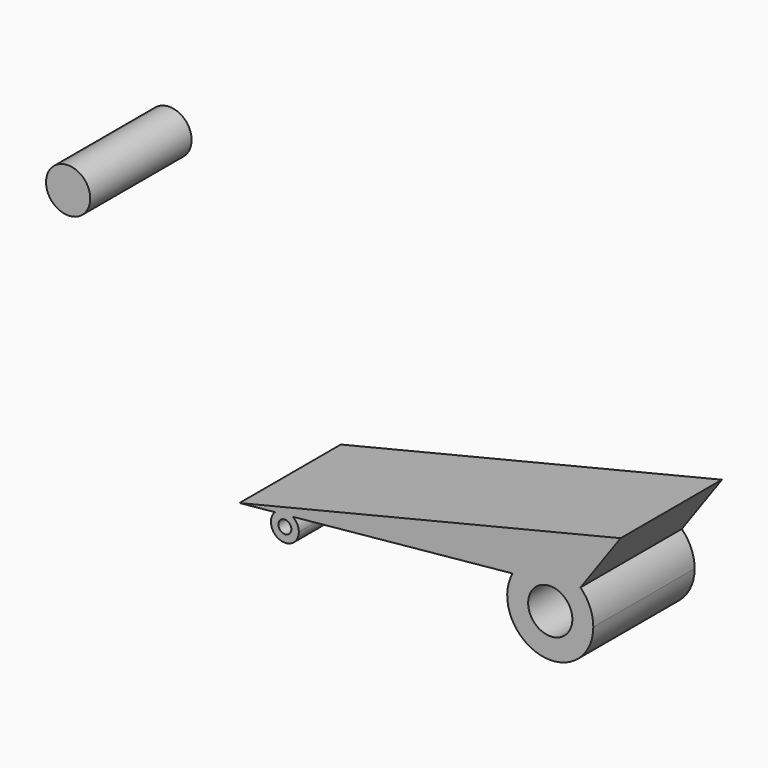
from build123d import *

# Parameters (mm, degrees)
F0_R     = 1.2955888687
F0_R_2   = 4.4335115967
F1_DEPTH = 25.4


with BuildPart() as f1:
    # F0 (on Front) → F1 (new body)
    with BuildSketch(Plane.XZ):
        with BuildLine():
            Line((89.1572237015, 31.5077528358), (12.7428583801, 12.8701059148))
            Line((12.7428583801, 12.8701059148), (19.8439891704, 13.5662951334))
            ThreePointArc((19.8439891704, 13.5662951334), (21.5718320787, 14.3954167349), (23.4278013561, 13.9176492317))
            Line((23.4278013561, 13.9176492317), (67.5118393184, 18.2396132754))
            ThreePointArc((67.5118393184, 18.2396132754), (73.8275336357, 22.5889714613), (81.112807161, 20.1952920757))
            Line((81.112807161, 20.1952920757), (89.1572237015, 31.5077528358))
        make_face()
        with BuildLine():
            ThreePointArc((23.4278013561, 13.9176492317), (21.5718320787, 14.3954167349), (19.8439891704, 13.5662951334))
            Line((19.8439891704, 13.5662951334), (23.4278013561, 13.9176492317))
        make_face()
        with BuildLine():
            Line((23.4278013561, 13.9176492317), (19.8439891704, 13.5662951334))
            ThreePointArc((19.8439891704, 13.5662951334), (20.7894933235, 9.0214762693), (24.6417307995, 11.6117702758))
            ThreePointArc((24.6417307995, 11.6117702758), (24.3197112814, 12.9147190903), (23.4278013561, 13.9176492317))
        make_face()
        with Locations((21.8447385651, 11.6117702758)):
            Circle(F0_R, mode=Mode.SUBTRACT)
        with BuildLine():
            ThreePointArc((83.6881530447, 14.0447923914), (83.0183282504, 17.3787484794), (81.112807161, 20.1952920757))
            Line((81.112807161, 20.1952920757), (80.6371569633, 19.5264089853))
            Line((80.6371569633, 19.5264089853), (67.5118393184, 18.2396132754))
            ThreePointArc((67.5118393184, 18.2396132754), (72.8893138351, 5.6891109706), (83.6881530447, 14.0447923914))
        make_face()
        with Locations((75.0560984015, 14.0447923914)):
            Circle(F0_R_2, mode=Mode.SUBTRACT)
        with BuildLine():
            Line((80.6371569633, 19.5264089853), (81.112807161, 20.1952920757))
            ThreePointArc((81.112807161, 20.1952920757), (73.8275336357, 22.5889714613), (67.5118393184, 18.2396132754))
            Line((67.5118393184, 18.2396132754), (80.6371569633, 19.5264089853))
        make_face()
    extrude(amount=F1_DEPTH)


with BuildPart() as f1b:
    # F0 (on Front) → F1, piece 2 (new body)
    with BuildSketch(Plane.XZ):
        with Locations((-21.6095242649, 56.8844042718)):
            Circle(F0_R_2)
    extrude(amount=F1_DEPTH)


solid = Compound([f1.part, f1b.part])
